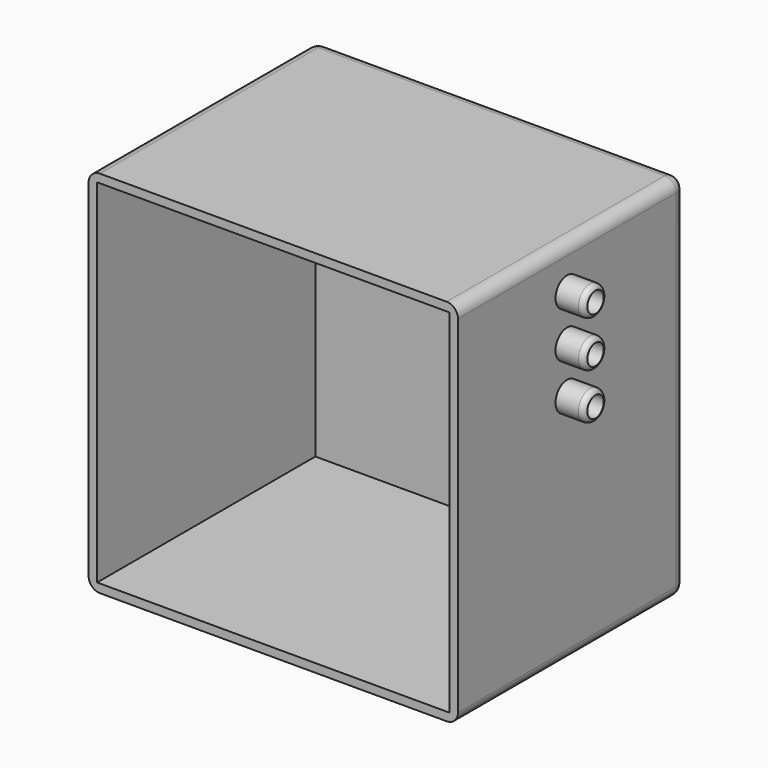
from build123d import *

# Parameters (mm, degrees)
F0_W     = 62
F0_H     = 62
F1_DEPTH = 2
F0_W_2   = 65
F0_H_2   = 65
F2_DEPTH = 50
F3_R     = 2
F4_R     = 1.8
F5_DEPTH = 25
F6_DEPTH = 25
F4_R_2   = 2.55
F7_DEPTH = 5


# Not quite as in the source:
# - a fillet or chamfer that OpenCascade refuses, or shapes differently, is made with other operations: its cross-section is extruded or revolved along the edge and cut away or added


with BuildPart() as f1:
    # F0 (on Front) → F1 (new body)
    with BuildSketch(Plane.XZ):
        with Locations((-0.6578962505, -3.6181825721)):
            Rectangle(F0_W, F0_H)
    extrude(amount=F1_DEPTH)

    # F0 (on Front) → F2 (join)
    with BuildSketch(Plane.XZ):
        with Locations((-0.6578962505, -3.6181825721)):
            Rectangle(F0_W_2, F0_H_2)
        with Locations((-0.6578962505, -3.6181825721)):
            Rectangle(F0_W, F0_H, mode=Mode.SUBTRACT)
    extrude(amount=F2_DEPTH)

    # F3
    f3_edges = [f1.edges().sort_by_distance(p)[0] for p in [
        (31.842104, 0, -3.618183),
        (-0.657896, 0, 28.881817),
        (-33.157896, 0, -3.618183),
        (-0.657896, 0, -36.118183),
        (31.842104, -25, 28.881817),
        (31.842104, -25, -36.118183),
        (-33.157896, -25, -36.118183),
        (-33.157896, -25, 28.881817),
    ]]
    fillet(f3_edges, radius=F3_R)

    # F4 (on face) → F5 (cut)
    with BuildSketch(Plane.YZ.offset(31.8421037495)):
        with Locations((-26, 21.3318174279)):
            Circle(F4_R)
    extrude(amount=-F5_DEPTH, mode=Mode.SUBTRACT)

    # F4 (on face) → F6 (cut)
    with BuildSketch(Plane.YZ.offset(31.8421037495)):
        with Locations((-26, 13.2318174279)):
            Circle(F4_R)
        with Locations((-26, 5.1318174279)):
            Circle(F4_R)
    extrude(amount=-F6_DEPTH, mode=Mode.SUBTRACT)

    # F4 (on face) → F7 (join)
    with BuildSketch(Plane.YZ.offset(31.8421037495)):
        with Locations((-26, 21.3318174279)):
            Circle(F4_R_2)
        with Locations((-26, 21.3318174279)):
            Circle(F4_R, mode=Mode.SUBTRACT)
        with Locations((-26, 13.2318174279)):
            Circle(F4_R_2)
        with Locations((-26, 13.2318174279)):
            Circle(F4_R, mode=Mode.SUBTRACT)
        with Locations((-26, 5.1318174279)):
            Circle(F4_R_2)
        with Locations((-26, 5.1318174279)):
            Circle(F4_R, mode=Mode.SUBTRACT)
    extrude(amount=F7_DEPTH)

    # F8: fillet of radius 1 on 3 edges, made by hand

    # F8_s1 → F8_t2 (revolve, cut)
    with BuildSketch(Plane.XY.offset(21.3318174279)):
        with BuildLine():
            ThreePointArc((35.873857913, -23.45), (36.4862303487, -23.659430585), (36.8421037495, -24.2))
            Line((36.8421037495, -24.2), (36.8421037495, -23.45))
            Line((36.8421037495, -23.45), (35.873857913, -23.45))
        make_face()
    revolve(axis=Axis((36.8421037495, -26, 21.3318174279), (1, 0, 0)), mode=Mode.SUBTRACT)

    # F8_s3 → F8_t4 (revolve, cut)
    with BuildSketch(Plane.XY.offset(13.2318174279)):
        with BuildLine():
            ThreePointArc((35.873857913, -23.45), (36.4862303487, -23.659430585), (36.8421037495, -24.2))
            Line((36.8421037495, -24.2), (36.8421037495, -23.45))
            Line((36.8421037495, -23.45), (35.873857913, -23.45))
        make_face()
    revolve(axis=Axis((36.8421037495, -26, 13.2318174279), (1, 0, 0)), mode=Mode.SUBTRACT)

    # F8_s5 → F8_t6 (revolve, cut)
    with BuildSketch(Plane.XY.offset(5.1318174279)):
        with BuildLine():
            ThreePointArc((35.873857913, -23.45), (36.4862303487, -23.659430585), (36.8421037495, -24.2))
            Line((36.8421037495, -24.2), (36.8421037495, -23.45))
            Line((36.8421037495, -23.45), (35.873857913, -23.45))
        make_face()
    revolve(axis=Axis((36.8421037495, -26, 5.1318174279), (1, 0, 0)), mode=Mode.SUBTRACT)


solid = f1.part
